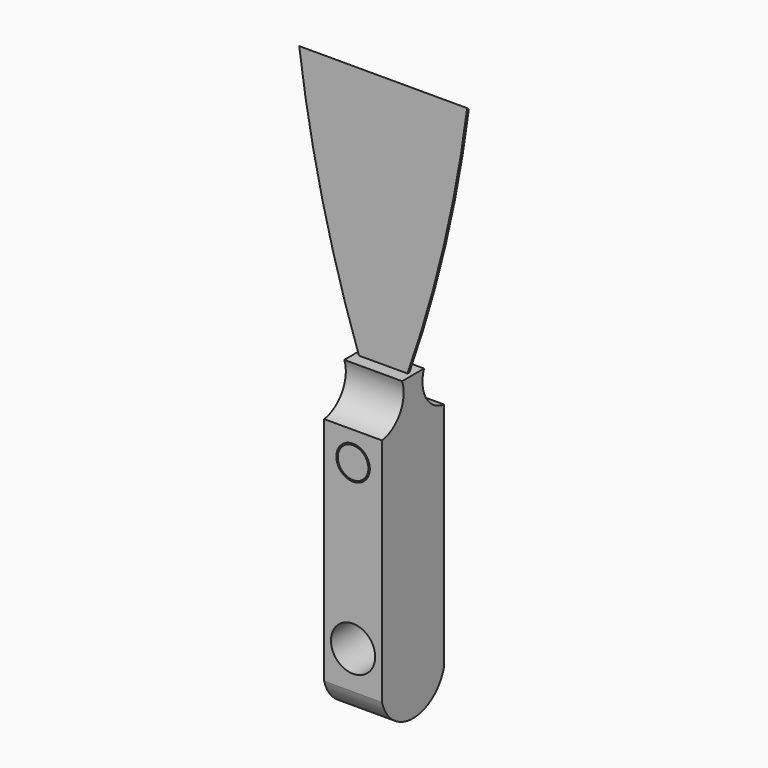
from build123d import *

# Parameters (mm, degrees)
F1_DEPTH    = 0.25
F3_DEPTH    = 6
F4_R        = 4.587200225
F5_DEPTH    = 17
F6_T1_DEPTH = 61.6245528892
F7_R        = 3.4767492544
F8_DEPTH    = 0.5
F9_R        = 3.1750599708
F10_DEPTH   = 0.5
F11_DEPTH   = 0.5


# Not quite as in the source:
# - a fillet or chamfer that OpenCascade refuses, or shapes differently, is made with other operations: its cross-section is extruded or revolved along the edge and cut away or added


with BuildPart() as f1:
    # F0 (on Front) → F1 (new body, symmetric)
    with BuildSketch(Plane.XZ):
        with BuildLine():
            Line((0, 44.4571785629), (-17.9538615048, 44.4571785629))
            ThreePointArc((-17.9538615048, 44.4571785629), (-13.1065795403, 15.5935304797), (-5.0346800126, -12.53920421))
            Line((-5.0346800126, -12.53920421), (0, -12.53920421))
            Line((0, -12.53920421), (0, 44.4571785629))
        make_face()
        with BuildLine():
            Line((17.9538615048, 44.4571785629), (0, 44.4571785629))
            Line((0, 44.4571785629), (0, -12.53920421))
            Line((0, -12.53920421), (5.0346800126, -12.53920421))
            ThreePointArc((5.0346800126, -12.53920421), (13.1065795403, 15.5935304797), (17.9538615048, 44.4571785629))
        make_face()
    extrude(amount=F1_DEPTH, both=True)

    # F6: chamfer of 5 on 1 edges, made by hand

    # F6_s2 → F6_t1 (cut)
    with BuildSketch(Plane.YZ.offset(-30.8122764446)):
        Polygon((-4.75, 44.4571785629), (0.25, 39.4571785629), (0.25, 44.4571785629), align=None)
    extrude(amount=F6_T1_DEPTH, mode=Mode.SUBTRACT)


with BuildPart() as f3:
    # F2 (on Right) → F3 (new body, symmetric)
    with BuildSketch(Plane.YZ):
        with BuildLine():
            Line((0, -12.5635201111), (-2.8466044459, -12.5635201111))
            ThreePointArc((-2.8466044459, -12.5635201111), (-3.3598513481, -18.1692156195), (-8.0613978207, -21.2648101151))
            Line((-8.0613978207, -21.2648101151), (-8.0613978207, -69.0904781222))
            ThreePointArc((-8.0613978207, -69.0904781222), (0, -75.2935267917), (8.0613978207, -69.0904781222))
            Line((8.0613978207, -69.0904781222), (8.0613978207, -21.2648101151))
            ThreePointArc((8.0613978207, -21.2648101151), (3.3598513481, -18.1692156195), (2.8466044459, -12.5635201111))
            Line((2.8466044459, -12.5635201111), (0, -12.5635201111))
        make_face()
    extrude(amount=F3_DEPTH, both=True)

    # F4 (on face) → F5 (cut)
    with BuildSketch(Plane.XZ.offset(8.0613978207)):
        with Locations((0, -61.2533651292)):
            Circle(F4_R)
    extrude(amount=-F5_DEPTH, mode=Mode.SUBTRACT)

    # F7 (on face) → F8 (cut)
    with BuildSketch(Plane.XZ.offset(8.0613978207)):
        with Locations((0, -27.280209586)):
            Circle(F7_R)
    extrude(amount=-F8_DEPTH, mode=Mode.SUBTRACT)

    # F9 (on face) → F10 (join)
    with BuildSketch(Plane.XZ.offset(7.5613978207)):
        with Locations((0, -27.280209586)):
            Circle(F9_R)
    extrude(amount=F10_DEPTH)

    # F9 (on face) → F11 (join)
    with BuildSketch(Plane.XZ.offset(7.5613978207)):
        with Locations((0, -27.280209586)):
            Circle(F9_R)
    extrude(amount=F11_DEPTH)


solid = Compound([f1.part, f3.part])
